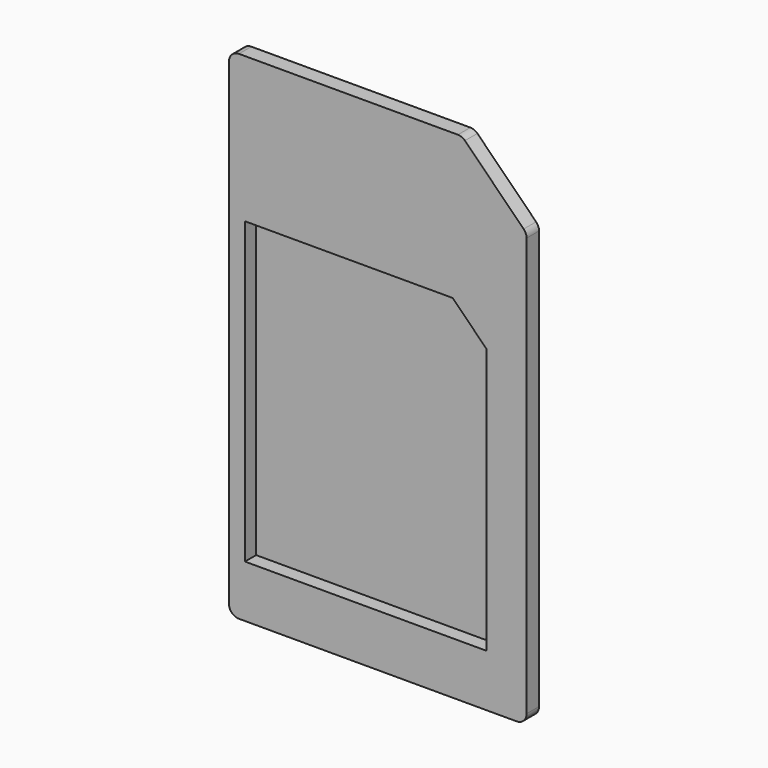
from build123d import *

# Parameters (mm, degrees)
F1_DEPTH = 0.78
F2_R     = 0.5
F4_DEPTH = 0.7


with BuildPart() as f1:
    # F0 (on Front) → F1 (new body)
    with BuildSketch(Plane.XZ):
        Polygon((4.2184664682, 12.45), (-7.45, 12.45), (-7.45, -12.45), (7.45, -12.45), (7.45, 9.2184664682), align=None)
    extrude(amount=F1_DEPTH)

    # F2
    f2_edges = [f1.edges().sort_by_distance(p)[0] for p in [
        (-7.45, -0.39, 12.45),
        (-7.45, -0.39, -12.45),
        (7.45, -0.39, -12.45),
        (7.45, -0.39, 9.218466),
        (4.218466, -0.39, 12.45),
    ]]
    fillet(f2_edges, radius=F2_R)

    # F3 (on face) → F4 (cut)
    with BuildSketch(Plane.XZ.offset(0.78)):
        Polygon((3.7478837054, 5.17), (-6.65, 5.17), (-6.65, -9.83), (5.45, -9.83), (5.45, 3.4678837054), align=None)
    extrude(amount=-F4_DEPTH, mode=Mode.SUBTRACT)


solid = f1.part
